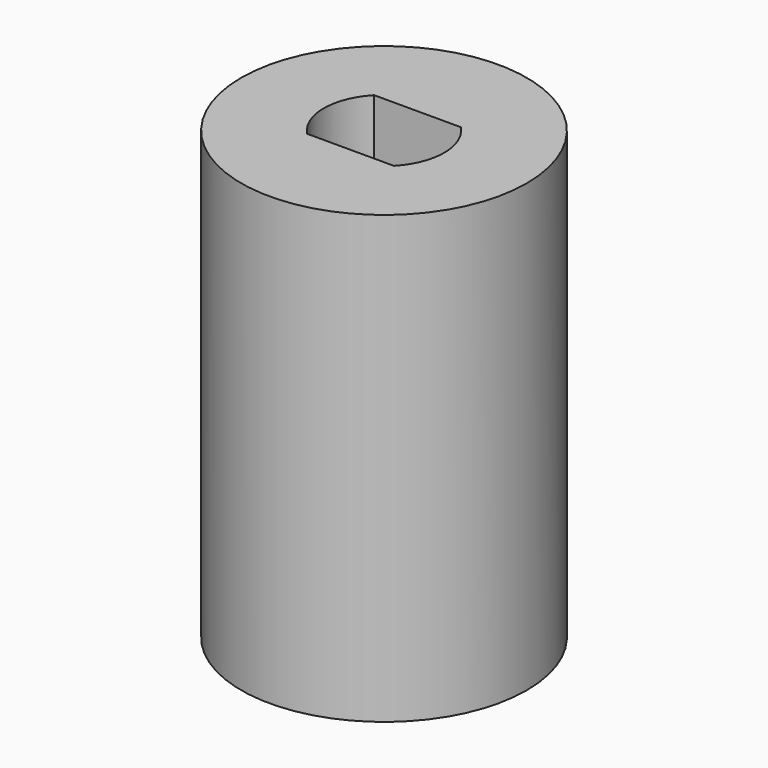
from build123d import *

# Parameters (mm, degrees)
F0_R     = 6.4
F1_DEPTH = 20
F3_DEPTH = 6
F4_R     = 2
F5_DEPTH = 14


# Not quite as in the source:
# - a feature names something its author has since deleted; it is built from what else it names


with BuildPart() as f1:
    # F0 (on Top) → F1 (new body)
    with BuildSketch(Plane.XY):
        Circle(F0_R)
    extrude(amount=F1_DEPTH)

    # F2 (on face) → F3 (cut)
    with BuildSketch(Plane.XY.offset(20)):
        with BuildLine():
            Line((1.942775077, 1.875), (-1.942775077, 1.875))
            ThreePointArc((-1.942775077, 1.875), (-2.7, 0), (-1.942775077, -1.875))
            Line((-1.942775077, -1.875), (1.942775077, -1.875))
            ThreePointArc((1.942775077, -1.875), (2.7, 0), (1.942775077, 1.875))
        make_face()
    extrude(amount=-F3_DEPTH, mode=Mode.SUBTRACT)

    # F4 (on face) → F5 (cut, through all)
    with BuildSketch(Plane(origin=(0, 0, 0), x_dir=(1, 0, 0), z_dir=(0, 0, -1))):
        Circle(F4_R)
    extrude(amount=-F5_DEPTH, mode=Mode.SUBTRACT)


solid = f1.part
